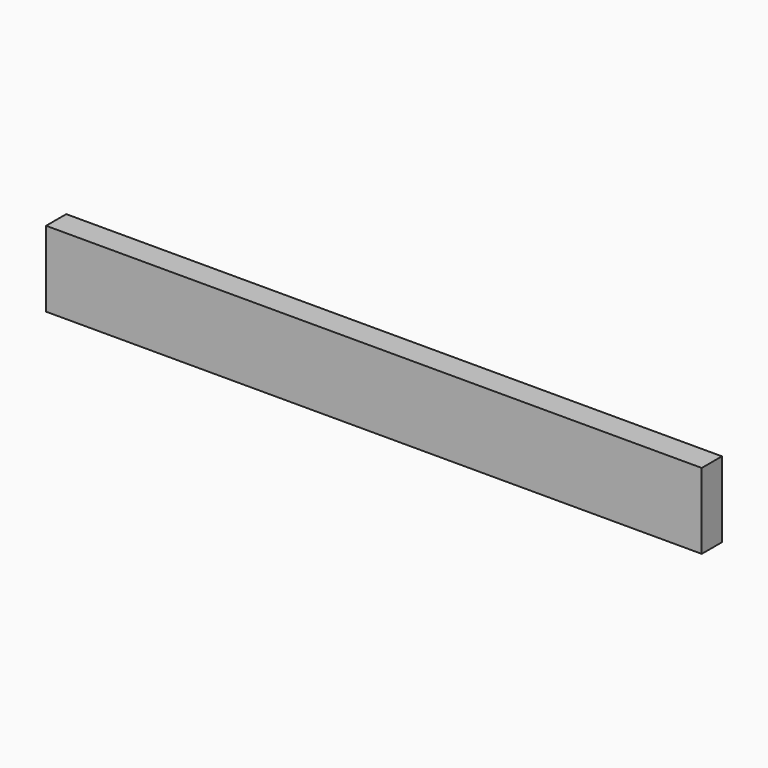
from build123d import *

# Parameters (mm, degrees)
F0_W     = 330.2
F0_H     = 38.1
F1_DEPTH = 12.7


# Not quite as in the source:
# - a feature names something its author has since deleted; it is built from what else it names


with BuildPart() as f1:
    # F0 (on Front) → F1 (new body)
    with BuildSketch(Plane.XZ):
        Rectangle(F0_W, F0_H)
    extrude(amount=F1_DEPTH)


solid = f1.part
